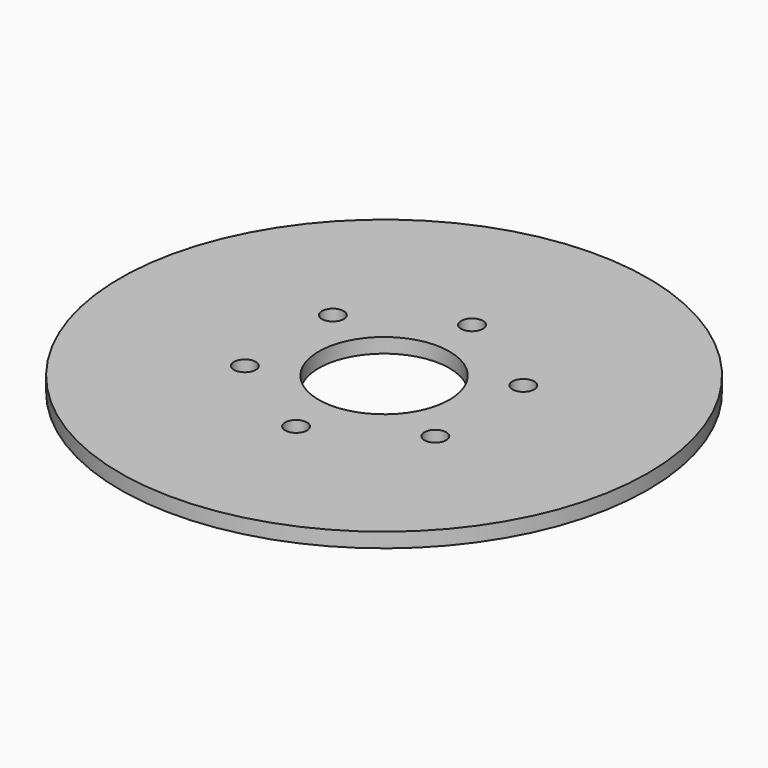
from build123d import *

# Parameters (mm, degrees)
F0_R            = 57.15
F0_R_2          = 14.1605
F1_DEPTH        = 3.175
F2_R            = 2.3622
F3_DEPTH        = 3.176
F3_COPIES_COUNT = 6


# Not quite as in the source:
# - a pattern or mirror of a feature is missing from the dataset's text; its kind, count and spacing are read off the source's solid


with BuildPart() as f1:
    # F0 (on Top) → F1 (new body)
    with BuildSketch(Plane.XY):
        Circle(F0_R)
        Circle(F0_R_2, mode=Mode.SUBTRACT)
    extrude(amount=F1_DEPTH)

    # F2 (on face) → F3 (cut, through all)
    with BuildSketch(Plane.XY.offset(3.175)):
        with Locations((0, 23.8125)):
            Circle(F2_R)
    f3 = extrude(amount=-F3_DEPTH, mode=Mode.SUBTRACT)

    # F3_copies: F3 ×6 about axis
    f3_copies_axis = Axis((0, 0, 0), (0, 0, 1))
    for i in range(1, F3_COPIES_COUNT):
        add(f3.rotate(f3_copies_axis, i * 360 / F3_COPIES_COUNT), mode=Mode.SUBTRACT)


solid = f1.part
